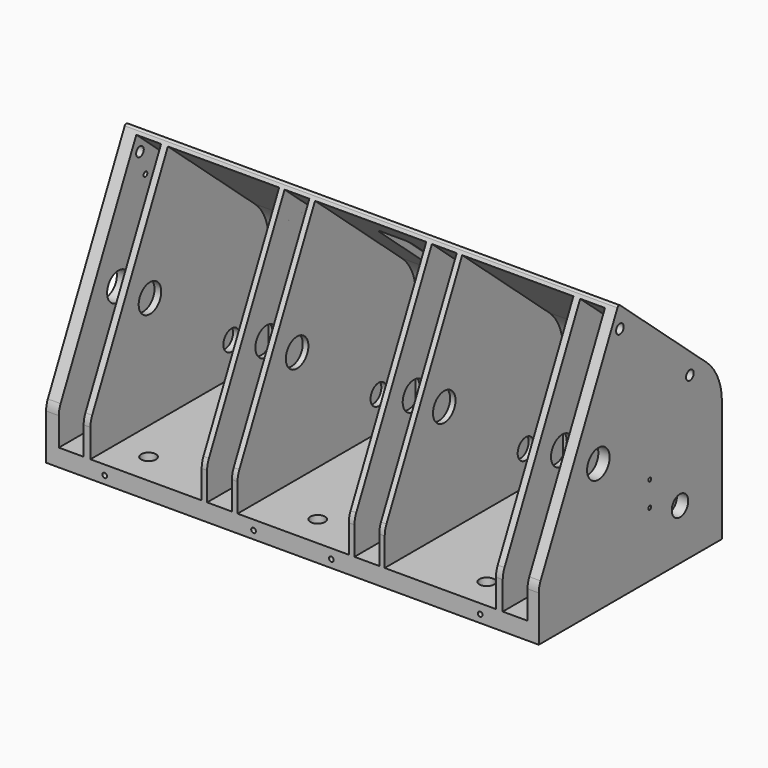
from build123d import *

# Parameters (mm, degrees)
F1_DEPTH         = 437
F3_START         = -10
F3_DEPTH         = 22
F4_START         = -38
F4_DEPTH         = 98.6666666667
F4_COPIES_COUNT  = 3
F4_COPIES_PITCH  = 130.500003
F5_START         = -141.5
F5_DEPTH         = 22
F6_START         = -168.5
F6_DEPTH         = 49.333335
F7_R             = 12.5
F7_R_2           = 9.1
F8_DEPTH         = 437.001
F11_D            = 3.3
F11_DEPTH        = 14.1
F11_TIP          = 0.9914200214
F12_D            = 4.2
F12_DEPTH        = 14.4
F12_TIP          = 1.2618073
F13_D            = 8.5
F13_DEPTH        = 15
F13_TIP          = 2.5536576309
F13_ON_F10_D     = 8.5
F13_ON_F10_DEPTH = 15
F13_ON_F10_TIP   = 2.5536576309
F15_D            = 4.2
F15_DEPTH        = 22.4
F15_TIP          = 1.2618073
F17_D            = 13
F17_DEPTH        = 20
F17_TIP          = 3.9055940237
F19_DEPTH        = 122


# Not quite as in the source:
# - a pattern or mirror of a feature is missing from the dataset's text; its kind, count and spacing are read off the source's solid


with BuildPart() as f1:
    # F0 (on Right) → F1 (new body)
    with BuildSketch(Plane.YZ):
        with BuildLine():
            Line((-203, 0), (0, 0))
            Line((0, 0), (0, 107.2598132073))
            ThreePointArc((0, 107.2598132073), (-4.4861055691, 127.9597024277), (-17.1394165495, 144.9451161156))
            Line((-17.1394165495, 144.9451161156), (-112.6975965799, 228.2693116758))
            ThreePointArc((-112.6975965799, 228.2693116758), (-114.4174744902, 228.7203700315), (-115.8168979667, 227.6235347659))
            Line((-115.8168979667, 227.6235347659), (-201.0487804878, 49.0872439281))
            ThreePointArc((-201.0487804878, 49.0872439281), (-202.5060966079, 44.8881529064), (-203, 40.4708918634))
            Line((-203, 40.4708918634), (-203, 0))
        make_face()
    extrude(amount=-F1_DEPTH)

    # F2 (on face) → F3 (cut)
    with BuildSketch(Plane.YZ.offset(F3_START)):
        with BuildLine():
            Line((-5.5, 15.5), (-5.5, 107.2598132073))
            ThreePointArc((-5.5, 107.2598132073), (-9.4926339565, 125.6827146135), (-20.754080729, 140.7997327957))
            Line((-20.754080729, 140.7997327957), (-121.0541861138, 228.258761349))
            Line((-121.0541861138, 228.258761349), (-205.5609756098, 51.2413319443))
            ThreePointArc((-205.5609756098, 51.2413319443), (-207.3826207599, 45.9924681672), (-208, 40.4708918634))
            Line((-208, 40.4708918634), (-208, 15.5))
            Line((-208, 15.5), (-197.5, 15.5))
            Line((-197.5, 15.5), (-5.5, 15.5))
        make_face()
    f3 = extrude(amount=-F3_DEPTH, mode=Mode.SUBTRACT)

    # F3_copies: F3 across plane
    add(f3.mirror(Plane(origin=(-152.083335, 0, 0), x_dir=(0, 0, -1), z_dir=(-1, 0, 0))), mode=Mode.SUBTRACT)

    # F3_copies1: F3 across plane
    add(f3.mirror(Plane(origin=(-217.833335, 0, 0), x_dir=(0, 0, -1), z_dir=(-1, 0, 0))), mode=Mode.SUBTRACT)

    # F2 (on face) → F4 (cut)
    with BuildSketch(Plane.YZ.offset(F4_START)):
        with BuildLine():
            Line((-5.5, 15.5), (-5.5, 107.2598132073))
            ThreePointArc((-5.5, 107.2598132073), (-9.4926339565, 125.6827146135), (-20.754080729, 140.7997327957))
            Line((-20.754080729, 140.7997327957), (-121.0541861138, 228.258761349))
            Line((-121.0541861138, 228.258761349), (-205.5609756098, 51.2413319443))
            ThreePointArc((-205.5609756098, 51.2413319443), (-207.3826207599, 45.9924681672), (-208, 40.4708918634))
            Line((-208, 40.4708918634), (-208, 15.5))
            Line((-208, 15.5), (-197.5, 15.5))
            Line((-197.5, 15.5), (-5.5, 15.5))
        make_face()
    f4 = extrude(amount=-F4_DEPTH, mode=Mode.SUBTRACT)

    # F4_copies: F4 ×3
    with Locations(*[(-i * F4_COPIES_PITCH, 0, 0) for i in range(1, F4_COPIES_COUNT)]):
        add(f4, mode=Mode.SUBTRACT)

    # F2 (on face) → F5 (cut)
    with BuildSketch(Plane.YZ.offset(F5_START)):
        with BuildLine():
            Line((-5.5, 15.5), (-5.5, 107.2598132073))
            ThreePointArc((-5.5, 107.2598132073), (-9.4926339565, 125.6827146135), (-20.754080729, 140.7997327957))
            Line((-20.754080729, 140.7997327957), (-121.0541861138, 228.258761349))
            Line((-121.0541861138, 228.258761349), (-205.5609756098, 51.2413319443))
            ThreePointArc((-205.5609756098, 51.2413319443), (-207.3826207599, 45.9924681672), (-208, 40.4708918634))
            Line((-208, 40.4708918634), (-208, 15.5))
            Line((-208, 15.5), (-197.5, 15.5))
            Line((-197.5, 15.5), (-5.5, 15.5))
        make_face()
    extrude(amount=-F5_DEPTH, mode=Mode.SUBTRACT)

    # F2 (on face) → F6 (cut)
    with BuildSketch(Plane.YZ.offset(F6_START)):
        with BuildLine():
            Line((-5.5, 15.5), (-5.5, 107.2598132073))
            ThreePointArc((-5.5, 107.2598132073), (-9.4926339565, 125.6827146135), (-20.754080729, 140.7997327957))
            Line((-20.754080729, 140.7997327957), (-121.0541861138, 228.258761349))
            Line((-121.0541861138, 228.258761349), (-205.5609756098, 51.2413319443))
            ThreePointArc((-205.5609756098, 51.2413319443), (-207.3826207599, 45.9924681672), (-208, 40.4708918634))
            Line((-208, 40.4708918634), (-208, 15.5))
            Line((-208, 15.5), (-197.5, 15.5))
            Line((-197.5, 15.5), (-5.5, 15.5))
        make_face()
    extrude(amount=-F6_DEPTH, mode=Mode.SUBTRACT)

    # F7 (on face) → F8 (cut, through all)
    with BuildSketch(Plane.YZ):
        with Locations((-137, 114.5)):
            Circle(F7_R)
        with Locations((-46.5, 45)):
            Circle(F7_R_2)
    extrude(amount=-F8_DEPTH, mode=Mode.SUBTRACT)

    # F11
    with Locations(Plane.YZ):
        with Locations((-80, 79), (-80, 57)):
            Hole(F11_D / 2, depth=F11_DEPTH)
            with Locations((0, 0, -(F11_DEPTH + F11_TIP / 2))):  # 118° drill point
                Cone(0, F11_D / 2, F11_TIP, mode=Mode.SUBTRACT)

    # F12
    with Locations(Plane(origin=(-437, 0, 0), x_dir=(0, -1, 0), z_dir=(-1, 0, 0))):
        with Locations((107, 190)):
            Hole(F12_D / 2, depth=F12_DEPTH)
            with Locations((0, 0, -(F12_DEPTH + F12_TIP / 2))):  # 118° drill point
                Cone(0, F12_D / 2, F12_TIP, mode=Mode.SUBTRACT)

    # F13
    with Locations(Plane(origin=(-437, 0, 0), x_dir=(0, -1, 0), z_dir=(-1, 0, 0))):
        with Locations((35.4877116727, 142.3694616976), (113.1194356637, 210.0622636058)):
            Hole(F13_D / 2, depth=F13_DEPTH)
            with Locations((0, 0, -(F13_DEPTH + F13_TIP / 2))):  # 118° drill point
                Cone(0, F13_D / 2, F13_TIP, mode=Mode.SUBTRACT)

    # F13 on F10
    with Locations(Plane.YZ):
        with Locations((-35.4877116727, 142.3694616976), (-113.1194356637, 210.0622636058)):
            Hole(F13_ON_F10_D / 2, depth=F13_ON_F10_DEPTH)
            with Locations((0, 0, -(F13_ON_F10_DEPTH + F13_ON_F10_TIP / 2))):  # 118° drill point
                Cone(0, F13_ON_F10_D / 2, F13_ON_F10_TIP, mode=Mode.SUBTRACT)

    # F15
    with Locations(Plane.XZ.offset(203)):
        with Locations((-385, 7), (-253, 7), (-184, 7), (-52, 7)):
            Hole(F15_D / 2, depth=F15_DEPTH)
            with Locations((0, 0, -(F15_DEPTH + F15_TIP / 2))):  # 118° drill point
                Cone(0, F15_D / 2, F15_TIP, mode=Mode.SUBTRACT)

    # F17
    with Locations(Plane(origin=(0, 0, 0), x_dir=(1, 0, 0), z_dir=(0, 0, -1))):
        with Locations((-368.5, 175), (-218.5, 175), (-68.5, 175), (-218.5, 63)):
            Hole(F17_D / 2, depth=F17_DEPTH)
            with Locations((0, 0, -(F17_DEPTH + F17_TIP / 2))):  # 118° drill point
                Cone(0, F17_D / 2, F17_TIP, mode=Mode.SUBTRACT)

    # F18 (on face) → F19 (cut)
    with BuildSketch(Plane(origin=(0, 0, 0), x_dir=(-1, 0, 0), z_dir=(0, 1, 0))):
        with BuildLine():
            Line((408.66667, 15.5), (420.66667, 15.5))
            ThreePointArc((420.66667, 15.5), (424.2022039059, 16.9644660941), (425.66667, 20.5))
            Line((425.66667, 20.5), (425.66667, 41.5))
            ThreePointArc((425.66667, 41.5), (424.2022039059, 45.0355339059), (420.66667, 46.5))
            Line((420.66667, 46.5), (408.66667, 46.5))
            ThreePointArc((408.66667, 46.5), (405.1311360941, 45.0355339059), (403.66667, 41.5))
            Line((403.66667, 41.5), (403.66667, 20.5))
            ThreePointArc((403.66667, 20.5), (405.1311360941, 16.9644660941), (408.66667, 15.5))
        make_face()
        with BuildLine():
            ThreePointArc((294.16667, 41.5), (292.8017413219, 44.9408397105), (289.4444466667, 46.5))
            Line((289.4444466667, 46.5), (277.4444466667, 46.5))
            ThreePointArc((277.4444466667, 46.5), (273.7279404156, 45.1374853404), (272.16667, 41.5))
            Line((272.16667, 41.5), (272.16667, 20.5))
            ThreePointArc((272.16667, 20.5), (273.6311360941, 16.9644660941), (277.16667, 15.5))
            Line((277.16667, 15.5), (289.16667, 15.5))
            ThreePointArc((289.16667, 15.5), (292.7022039059, 16.9644660941), (294.16667, 20.5))
            Line((294.16667, 20.5), (294.16667, 41.5))
        make_face()
        with BuildLine():
            ThreePointArc((163.5, 41.5), (161.9387295844, 45.1374853404), (158.2222233333, 46.5))
            Line((158.2222233333, 46.5), (146.2222233333, 46.5))
            ThreePointArc((146.2222233333, 46.5), (142.8649286781, 44.9408397105), (141.5, 41.5))
            Line((141.5, 41.5), (141.5, 20.5))
            ThreePointArc((141.5, 20.5), (142.8649286781, 17.0591602895), (146.2222233333, 15.5))
            Line((146.2222233333, 15.5), (158.5, 15.5))
            ThreePointArc((158.5, 15.5), (162.0355339059, 16.9644660941), (163.5, 20.5))
            Line((163.5, 20.5), (163.5, 41.5))
        make_face()
        with BuildLine():
            ThreePointArc((32, 41.5), (30.5355339059, 45.0355339059), (27, 46.5))
            Line((27, 46.5), (15, 46.5))
            ThreePointArc((15, 46.5), (11.4644660941, 45.0355339059), (10, 41.5))
            Line((10, 41.5), (10, 20.5))
            ThreePointArc((10, 20.5), (11.4644660941, 16.9644660941), (15, 15.5))
            Line((15, 15.5), (27, 15.5))
            ThreePointArc((27, 15.5), (30.5355339059, 16.9644660941), (32, 20.5))
            Line((32, 20.5), (32, 41.5))
        make_face()
        with BuildLine():
            ThreePointArc((425.66667, 199), (424.2022039059, 202.5355339059), (420.66667, 204))
            Line((420.66667, 204), (408.66667, 204))
            ThreePointArc((408.66667, 204), (405.1311360941, 202.5355339059), (403.66667, 199))
            Line((403.66667, 199), (403.66667, 159))
            ThreePointArc((403.66667, 159), (405.1311360941, 155.4644660941), (408.66667, 154))
            Line((408.66667, 154), (420.66667, 154))
            ThreePointArc((420.66667, 154), (424.2022039059, 155.4644660941), (425.66667, 159))
            Line((425.66667, 159), (425.66667, 199))
        make_face()
        with BuildLine():
            ThreePointArc((294.16667, 199), (292.8017413219, 202.4408397105), (289.4444466667, 204))
            Line((289.4444466667, 204), (277.4444466667, 204))
            ThreePointArc((277.4444466667, 204), (273.7279404156, 202.6374853404), (272.16667, 199))
            Line((272.16667, 199), (272.16667, 159))
            ThreePointArc((272.16667, 159), (273.6311360941, 155.4644660941), (277.16667, 154))
            Line((277.16667, 154), (289.16667, 154))
            ThreePointArc((289.16667, 154), (292.7022039059, 155.4644660941), (294.16667, 159))
            Line((294.16667, 159), (294.16667, 199))
        make_face()
        with BuildLine():
            ThreePointArc((163.5, 199), (162.0355339059, 202.5355339059), (158.5, 204))
            Line((158.5, 204), (146.5, 204))
            ThreePointArc((146.5, 204), (142.9644660941, 202.5355339059), (141.5, 199))
            Line((141.5, 199), (141.5, 159))
            ThreePointArc((141.5, 159), (142.9644660941, 155.4644660941), (146.5, 154))
            Line((146.5, 154), (158.5, 154))
            ThreePointArc((158.5, 154), (162.0355339059, 155.4644660941), (163.5, 159))
            Line((163.5, 159), (163.5, 199))
        make_face()
        with BuildLine():
            ThreePointArc((32, 199), (30.5355339059, 202.5355339059), (27, 204))
            Line((27, 204), (15, 204))
            ThreePointArc((15, 204), (11.4644660941, 202.5355339059), (10, 199))
            Line((10, 199), (10, 159))
            ThreePointArc((10, 159), (11.4644660941, 155.4644660941), (15, 154))
            Line((15, 154), (27, 154))
            ThreePointArc((27, 154), (30.5355339059, 155.4644660941), (32, 159))
            Line((32, 159), (32, 199))
        make_face()
        with BuildLine():
            Line((227.55667, 204), (207.55667, 204))
            ThreePointArc((207.55667, 204), (204.0211360941, 202.5355339059), (202.55667, 199))
            Line((202.55667, 199), (202.55667, 159))
            ThreePointArc((202.55667, 159), (204.0211360941, 155.4644660941), (207.55667, 154))
            Line((207.55667, 154), (227.55667, 154))
            ThreePointArc((227.55667, 154), (231.0922039059, 155.4644660941), (232.55667, 159))
            Line((232.55667, 159), (232.55667, 199))
            ThreePointArc((232.55667, 199), (231.0922039059, 202.5355339059), (227.55667, 204))
        make_face()
    extrude(amount=-F19_DEPTH, mode=Mode.SUBTRACT)


solid = f1.part
